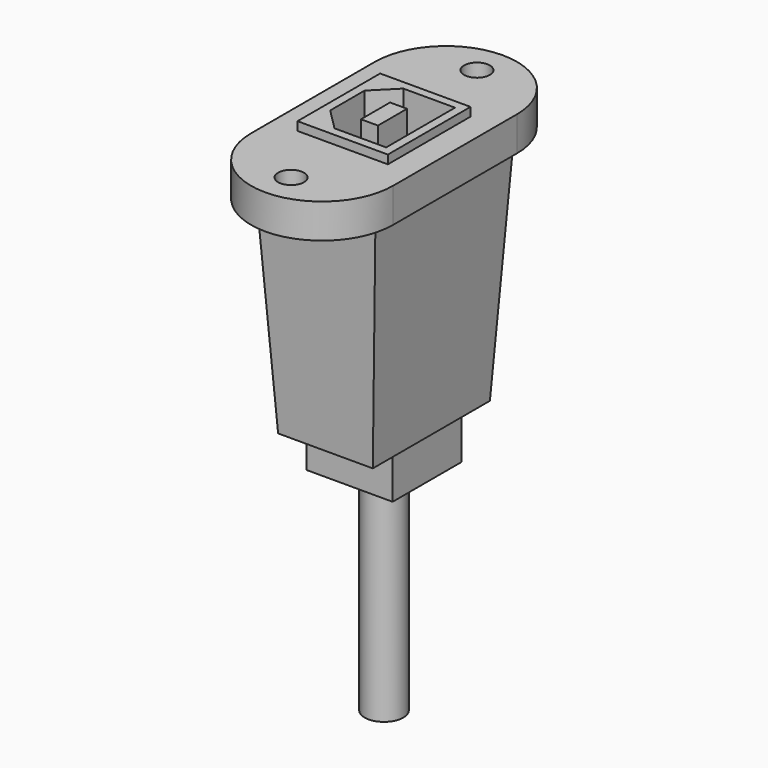
from build123d import *

# Parameters (mm, degrees)
F0_R      = 1.5
F1_DEPTH  = 4
F2_W      = 14
F2_H      = 20
F3_DEPTH  = 26
F4_SIZE2  = 25.99999
F4_SIZE   = 1.49999
F5_W      = 10
F5_H      = 10
F6_DEPTH  = 5
F7_R      = 2.25
F8_DEPTH  = 25
F9_DEPTH  = 18
F10_W     = 10.5
F10_H     = 12
F11_DEPTH = 1
F13_W     = 8.5
F13_H     = 10
F13_W_2   = 1.9773303065
F13_H_2   = 4.2267278768
F14_DEPTH = 5
F15_SIZE  = 2.5


# Not quite as in the source:
# - a fillet or chamfer is up to 0.001 mm smaller than in the source, because OpenCascade refuses the exact size
# - a feature names something its author has since deleted; it is built from what else it names


with BuildPart() as f1:
    # F0 (on Top) → F1 (new body)
    with BuildSketch(Plane.XY):
        with BuildLine():
            Line((-8.25, 9), (8.25, 9))
            ThreePointArc((8.25, 9), (0, 17.25), (-8.25, 9))
        make_face()
        with Locations((0, 13.5)):
            Circle(F0_R, mode=Mode.SUBTRACT)
    extrude(amount=-F1_DEPTH)



with BuildPart() as f1b:
    # F0 (on Top) → F1, piece 2 (new body)
    with BuildSketch(Plane.XY):
        with BuildLine():
            ThreePointArc((-8.25, -9), (0, -17.25), (8.25, -9))
            Line((8.25, -9), (-8.25, -9))
        make_face()
        with Locations((0, -13.5)):
            Circle(F0_R, mode=Mode.SUBTRACT)
    extrude(amount=-F1_DEPTH)


with BuildPart() as f1_1:
    add(f1.part)

    add(f1b.part)  # F3 merges F1b
    # F2 (on face) → F3 (join)
    with BuildSketch(Plane(origin=(0, 0, -4), x_dir=(1, 0, 0), z_dir=(0, 0, -1))):
        Rectangle(F2_W, F2_H)
    extrude(amount=F3_DEPTH)

    # F4 (size 1.5 and 26 in the source; OpenCascade refuses exactly that, so slightly less here)
    f4_edges = [f1_1.edges().sort_by_distance(p)[0] for p in [
        (0, -10, -30),
        (0, 10, -30),
        (7, 0, -30),
        (-7, 0, -30),
    ]]
    f4_side = f1_1.faces().sort_by_distance((0, 0, -30))[0]
    chamfer(f4_edges, length=F4_SIZE, length2=F4_SIZE2, reference=f4_side)

    # F5 (on face) → F6 (join)
    with BuildSketch(Plane(origin=(0, 0, -30), x_dir=(1, 0, 0), z_dir=(0, 0, -1))):
        Rectangle(F5_W, F5_H)
    extrude(amount=F6_DEPTH)

    # F7 (on face) → F8 (join)
    with BuildSketch(Plane(origin=(0, 0, -35), x_dir=(1, 0, 0), z_dir=(0, 0, -1))):
        Circle(F7_R)
    extrude(amount=F8_DEPTH)

    # F9 (add): a face of the model
    f9_faces = [f1_1.faces().sort_by_distance(p)[0] for p in [
        (0, -9, -2),
    ]]
    extrude(f9_faces, amount=F9_DEPTH)

    # F10 (on face) → F11 (join)
    with BuildSketch(Plane.XY):
        Rectangle(F10_W, F10_H)
    extrude(amount=F11_DEPTH)

    # F13 (on face) → F14 (cut)
    with BuildSketch(Plane.XY.offset(1)):
        Rectangle(F13_W, F13_H)
        Rectangle(F13_W_2, F13_H_2, mode=Mode.SUBTRACT)
    extrude(amount=-F14_DEPTH, mode=Mode.SUBTRACT)

    # F15
    f15_edges = [f1_1.edges().sort_by_distance(p)[0] for p in [
        (-4.25, -5, -1.5),
        (-4.25, 5, -1.5),
    ]]
    chamfer(f15_edges, length=F15_SIZE)


solid = f1_1.part
